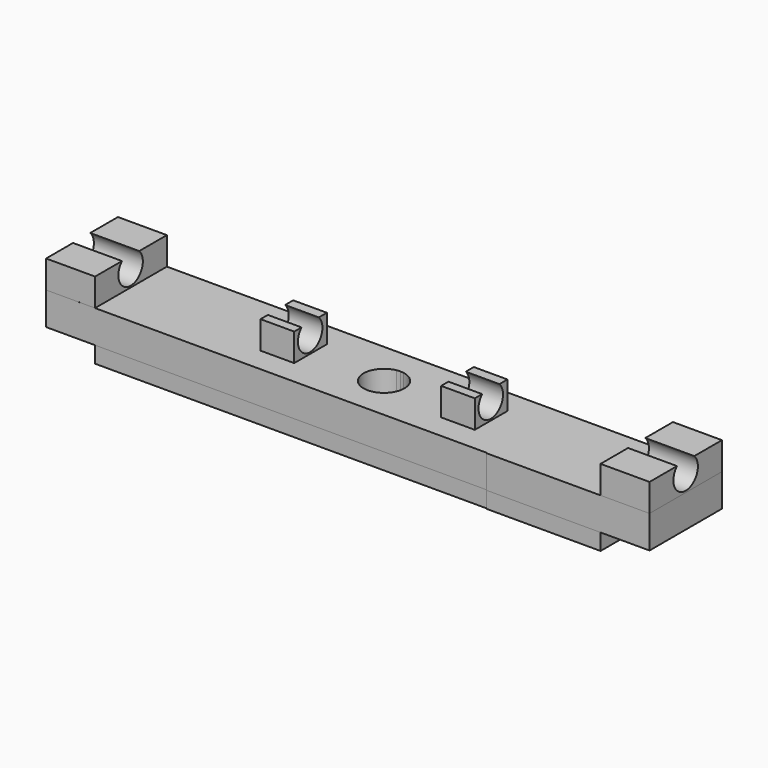
from build123d import *

# Parameters (mm, degrees)
F0_W          = 17.78
F0_H          = 13.97
F1_DEPTH      = 2.54
F2_START      = 2.54
F0_W_2        = 7.62
F0_H_2        = 14.0794469044
F2_DEPTH      = 5.08
F3_START      = 7.62
F3_DEPTH      = 4.318
F4_R          = 2.38125
F5_DEPTH      = 50.8
F5_DEPTH_BACK = 50.8


with BuildPart() as f1:
    # F0 (on Top) → F1 (new body)
    with BuildSketch(Plane.XY):
        Polygon((-21.0799529247, 0), (-21.0799529247, -13.97), (-10.9199529247, -13.97), (-10.9199529247, -10.16), (-16.1587029247, -10.16), (-16.1587029247, -8.7376), (-16.1587029247, -5.2451), (-16.1587029247, -3.81), (-10.9199529247, -3.81), (-10.9199529247, 0), align=None)
        with Locations((-29.9699529247, -6.985)):
            Rectangle(F0_W, F0_H)
        Polygon((-10.9199529247, -10.16), (-10.9199529247, -13.97), (11.9400470753, -13.97), (11.9400470753, -10.16), (0.5100470753, -10.16), align=None)
        Polygon((11.9400470753, -10.16), (11.9400470753, -13.97), (22.1000470753, -13.97), (22.1000470753, 0), (11.9400470753, 0), (11.9400470753, -3.81), (17.1787970753, -3.81), (17.1787970753, -5.2324), (17.1787970753, -8.7376), (17.1787970753, -10.16), align=None)
        with BuildLine():
            Line((-10.9199529247, -9.1745346656), (-10.9199529247, -10.16))
            Line((-10.9199529247, -10.16), (0.5100470753, -10.16))
            ThreePointArc((0.5100470753, -10.16), (0.1173051299, -10.1356156167), (-0.2694042043, -10.0628370169))
            Line((-0.2694042043, -10.0628370169), (-10.9199529247, -9.1745346656))
        make_face()
        Polygon((-16.1587029247, -10.16), (-10.9199529247, -10.16), (-10.9199529247, -9.1745346656), (-16.1587029247, -8.7376), align=None)
        Polygon((11.9400470753, 0), (-10.9199529247, 0), (-10.9199529247, -3.81), (0.5100470753, -3.81), (11.9400470753, -3.81), align=None)
        Polygon((22.1000470753, 0), (22.1000470753, -13.97), (22.1000470753, -14.0794469044), (39.8800470753, -14.0794469044), (39.8800470753, 0), align=None)
        Polygon((11.9400470753, -9.1745346656), (11.9400470753, -10.16), (17.1787970753, -10.16), (17.1787970753, -8.7376), align=None)
        with BuildLine():
            Line((0.5100470753, -10.16), (11.9400470753, -10.16))
            Line((11.9400470753, -10.16), (11.9400470753, -9.1745346656))
            Line((11.9400470753, -9.1745346656), (1.2894983548, -10.0628370169))
            ThreePointArc((1.2894983548, -10.0628370169), (0.9027890206, -10.1356156167), (0.5100470753, -10.16))
        make_face()
        Polygon((-10.9199529247, -4.7940685714), (-10.9199529247, -3.81), (-16.1587029247, -3.81), (-16.1587029247, -5.2451), align=None)
        with BuildLine():
            Line((0.5100470753, -3.81), (-10.9199529247, -3.81))
            Line((-10.9199529247, -3.81), (-10.9199529247, -4.7940685714))
            Line((-10.9199529247, -4.7940685714), (-0.0326351146, -3.8567223523))
            ThreePointArc((-0.0326351146, -3.8567223523), (0.237702194, -3.8217021535), (0.5100470753, -3.81))
        make_face()
        with BuildLine():
            Line((11.9400470753, -4.78536), (11.9400470753, -3.81))
            Line((11.9400470753, -3.81), (0.5100470753, -3.81))
            ThreePointArc((0.5100470753, -3.81), (0.7799993252, -3.8214970708), (1.0479965137, -3.8559050187))
            Line((1.0479965137, -3.8559050187), (11.9400470753, -4.78536))
        make_face()
        Polygon((17.1787970753, -3.81), (11.9400470753, -3.81), (11.9400470753, -4.78536), (17.1787970753, -5.2324), align=None)
    extrude(amount=F1_DEPTH)


with BuildPart() as f2:
    # F0 (on Top) → F2 (new body)
    with BuildSketch(Plane.XY.offset(F2_START)):
        Polygon((-21.0799529247, 0), (-21.0799529247, -13.97), (-10.9199529247, -13.97), (-10.9199529247, -10.16), (-16.1587029247, -10.16), (-16.1587029247, -8.7376), (-16.1587029247, -5.2451), (-16.1587029247, -3.81), (-10.9199529247, -3.81), (-10.9199529247, 0), align=None)
        with Locations((-29.9699529247, -6.985)):
            Rectangle(F0_W, F0_H)
        Polygon((-10.9199529247, -10.16), (-10.9199529247, -13.97), (11.9400470753, -13.97), (11.9400470753, -10.16), (0.5100470753, -10.16), align=None)
        with Locations((-42.6699529247, -6.985)):
            Rectangle(F0_W_2, F0_H)
        Polygon((11.9400470753, -10.16), (11.9400470753, -13.97), (22.1000470753, -13.97), (22.1000470753, 0), (11.9400470753, 0), (11.9400470753, -3.81), (17.1787970753, -3.81), (17.1787970753, -5.2324), (17.1787970753, -8.7376), (17.1787970753, -10.16), align=None)
        with BuildLine():
            Line((-10.9199529247, -9.1745346656), (-10.9199529247, -10.16))
            Line((-10.9199529247, -10.16), (0.5100470753, -10.16))
            ThreePointArc((0.5100470753, -10.16), (0.1173051299, -10.1356156167), (-0.2694042043, -10.0628370169))
            Line((-0.2694042043, -10.0628370169), (-10.9199529247, -9.1745346656))
        make_face()
        Polygon((-16.1587029247, -10.16), (-10.9199529247, -10.16), (-10.9199529247, -9.1745346656), (-16.1587029247, -8.7376), align=None)
        Polygon((11.9400470753, 0), (-10.9199529247, 0), (-10.9199529247, -3.81), (0.5100470753, -3.81), (11.9400470753, -3.81), align=None)
        Polygon((22.1000470753, 0), (22.1000470753, -13.97), (22.1000470753, -14.0794469044), (39.8800470753, -14.0794469044), (39.8800470753, 0), align=None)
        Polygon((11.9400470753, -9.1745346656), (11.9400470753, -10.16), (17.1787970753, -10.16), (17.1787970753, -8.7376), align=None)
        with BuildLine():
            Line((0.5100470753, -10.16), (11.9400470753, -10.16))
            Line((11.9400470753, -10.16), (11.9400470753, -9.1745346656))
            Line((11.9400470753, -9.1745346656), (1.2894983548, -10.0628370169))
            ThreePointArc((1.2894983548, -10.0628370169), (0.9027890206, -10.1356156167), (0.5100470753, -10.16))
        make_face()
        with BuildLine():
            Line((-10.9199529247, -4.7940685714), (-10.9199529247, -9.1745346656))
            Line((-10.9199529247, -9.1745346656), (-0.2694042043, -10.0628370169))
            ThreePointArc((-0.2694042043, -10.0628370169), (-2.6626448473, -6.8639588303), (-0.0326351146, -3.8567223523))
            Line((-0.0326351146, -3.8567223523), (-10.9199529247, -4.7940685714))
        make_face()
        Polygon((-16.1587029247, -8.7376), (-10.9199529247, -9.1745346656), (-10.9199529247, -4.7940685714), (-16.1587029247, -5.2451), align=None)
        Polygon((-10.9199529247, -4.7940685714), (-10.9199529247, -3.81), (-16.1587029247, -3.81), (-16.1587029247, -5.2451), align=None)
        with BuildLine():
            Line((0.5100470753, -3.81), (-10.9199529247, -3.81))
            Line((-10.9199529247, -3.81), (-10.9199529247, -4.7940685714))
            Line((-10.9199529247, -4.7940685714), (-0.0326351146, -3.8567223523))
            ThreePointArc((-0.0326351146, -3.8567223523), (0.237702194, -3.8217021535), (0.5100470753, -3.81))
        make_face()
        Polygon((11.9400470753, -4.78536), (11.9400470753, -9.1745346656), (17.1787970753, -8.7376), (17.1787970753, -5.2324), align=None)
        with BuildLine():
            Line((1.2894983548, -10.0628370169), (11.9400470753, -9.1745346656))
            Line((11.9400470753, -9.1745346656), (11.9400470753, -4.78536))
            Line((11.9400470753, -4.78536), (1.0479965137, -3.8559050187))
            ThreePointArc((1.0479965137, -3.8559050187), (2.9378665153, -4.938950693), (3.6850470753, -6.985))
            ThreePointArc((3.6850470753, -6.985), (3.0155792356, -8.9351111747), (1.2894983548, -10.0628370169))
        make_face()
        with BuildLine():
            Line((11.9400470753, -4.78536), (11.9400470753, -3.81))
            Line((11.9400470753, -3.81), (0.5100470753, -3.81))
            ThreePointArc((0.5100470753, -3.81), (0.7799993252, -3.8214970708), (1.0479965137, -3.8559050187))
            Line((1.0479965137, -3.8559050187), (11.9400470753, -4.78536))
        make_face()
        Polygon((17.1787970753, -3.81), (11.9400470753, -3.81), (11.9400470753, -4.78536), (17.1787970753, -5.2324), align=None)
        with Locations((43.6900470753, -7.0397234522)):
            Rectangle(F0_W_2, F0_H_2)
    extrude(amount=F2_DEPTH)


with BuildPart() as f3:
    # F0 (on Top) → F3 (new body)
    with BuildSketch(Plane.XY.offset(F3_START)):
        Polygon((-16.1587029247, -10.16), (-10.9199529247, -10.16), (-10.9199529247, -9.1745346656), (-16.1587029247, -8.7376), align=None)
        Polygon((-10.9199529247, -4.7940685714), (-10.9199529247, -3.81), (-16.1587029247, -3.81), (-16.1587029247, -5.2451), align=None)
        Polygon((-16.1587029247, -8.7376), (-10.9199529247, -9.1745346656), (-10.9199529247, -4.7940685714), (-16.1587029247, -5.2451), align=None)
    extrude(amount=F3_DEPTH)


with BuildPart() as f3b:
    # F0 (on Top) → F3, piece 2 (new body)
    with BuildSketch(Plane.XY.offset(F3_START)):
        Polygon((17.1787970753, -3.81), (11.9400470753, -3.81), (11.9400470753, -4.78536), (17.1787970753, -5.2324), align=None)
        Polygon((11.9400470753, -4.78536), (11.9400470753, -9.1745346656), (17.1787970753, -8.7376), (17.1787970753, -5.2324), align=None)
        Polygon((11.9400470753, -9.1745346656), (11.9400470753, -10.16), (17.1787970753, -10.16), (17.1787970753, -8.7376), align=None)
    extrude(amount=F3_DEPTH)


with BuildPart() as f3c:
    # F0 (on Top) → F3, piece 3 (new body)
    with BuildSketch(Plane.XY.offset(F3_START)):
        with Locations((-42.6699529247, -6.985)):
            Rectangle(F0_W_2, F0_H)
    extrude(amount=F3_DEPTH)


with BuildPart() as f3d:
    # F0 (on Top) → F3, piece 4 (new body)
    with BuildSketch(Plane.XY.offset(F3_START)):
        with Locations((43.6900470753, -7.0397234522)):
            Rectangle(F0_W_2, F0_H_2)
    extrude(amount=F3_DEPTH)


with BuildPart() as f5_tool:
    # F4 (on Right) → F5 (new body, two sides)
    with BuildSketch(Plane.YZ) as f5_sk:
        with Locations((-7.0559619926, 10.248853825)):
            Circle(F4_R)
    extrude(amount=-F5_DEPTH)
    extrude(f5_sk.sketch, amount=F5_DEPTH_BACK)


with BuildPart() as f3_1:
    add(f3.part)

    # F5: cut by f5_tool
    add(f5_tool.part, mode=Mode.SUBTRACT)


with BuildPart() as f3b_1:
    add(f3b.part)

    # F5: cut by f5_tool
    add(f5_tool.part, mode=Mode.SUBTRACT)


with BuildPart() as f3c_1:
    add(f3c.part)

    # F5: cut by f5_tool
    add(f5_tool.part, mode=Mode.SUBTRACT)


with BuildPart() as f3d_1:
    add(f3d.part)

    # F5: cut by f5_tool
    add(f5_tool.part, mode=Mode.SUBTRACT)


solid = Compound([f1.part, f2.part, f3_1.part, f3b_1.part, f3c_1.part, f3d_1.part])
